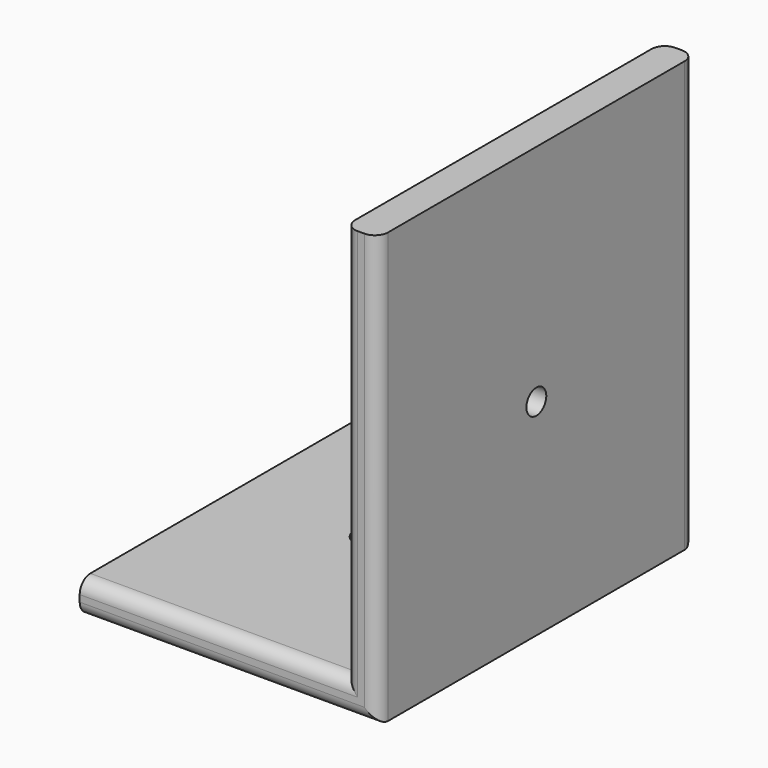
from build123d import *

# Parameters (mm, degrees)
F1_DEPTH = 152.4
F3_D     = 9.525
F5_D     = 12.7
F6_R     = 5.08
F7_R     = 5.08
F8_R     = 5.08
F9_R     = 5.08


# Not quite as in the source:
# - a length typed as a fraction of an inch, garbled in the dataset ("3 / 203.2 mm" for 3/8 in), is restored


with BuildPart() as f1:
    # F0 (on Front) → F1 (new body)
    with BuildSketch(Plane.XZ):
        Polygon((0, -78.9952108244), (0, 86.1047891756), (-12.7, 86.1047891756), (-12.7, -66.2952108244), (-114.3, -66.2952108244), (-114.3, -78.9952108244), align=None)
    extrude(amount=F1_DEPTH)

    # F3 (through all)
    with Locations(Plane.YZ):
        with Locations((-76.2, 0)):
            Hole(F3_D / 2)

    # F5 (through all)
    with Locations(Plane.XY.offset(-66.2952108244)):
        with Locations((-63.5, -76.2)):
            Hole(F5_D / 2)

    # F6
    f6_edges = [f1.edges().sort_by_distance(p)[0] for p in [
        (-12.7, -152.4, 9.904789),
        (-63.5, -152.4, -66.295211),
    ]]
    fillet(f6_edges, radius=F6_R)

    # F7
    f7_edges = [f1.edges().sort_by_distance(p)[0] for p in [
        (-12.7, 0, 9.904789),
        (-63.5, 0, -66.295211),
    ]]
    fillet(f7_edges, radius=F7_R)

    # F8
    f8_edges = [f1.edges().sort_by_distance(p)[0] for p in [
        (-57.15, 0, -78.995211),
        (0, 0, 3.554789),
    ]]
    fillet(f8_edges, radius=F8_R)

    # F9
    f9_edges = [f1.edges().sort_by_distance(p)[0] for p in [
        (-57.15, -152.4, -78.995211),
        (0, -152.4, 3.554789),
    ]]
    fillet(f9_edges, radius=F9_R)


solid = f1.part
